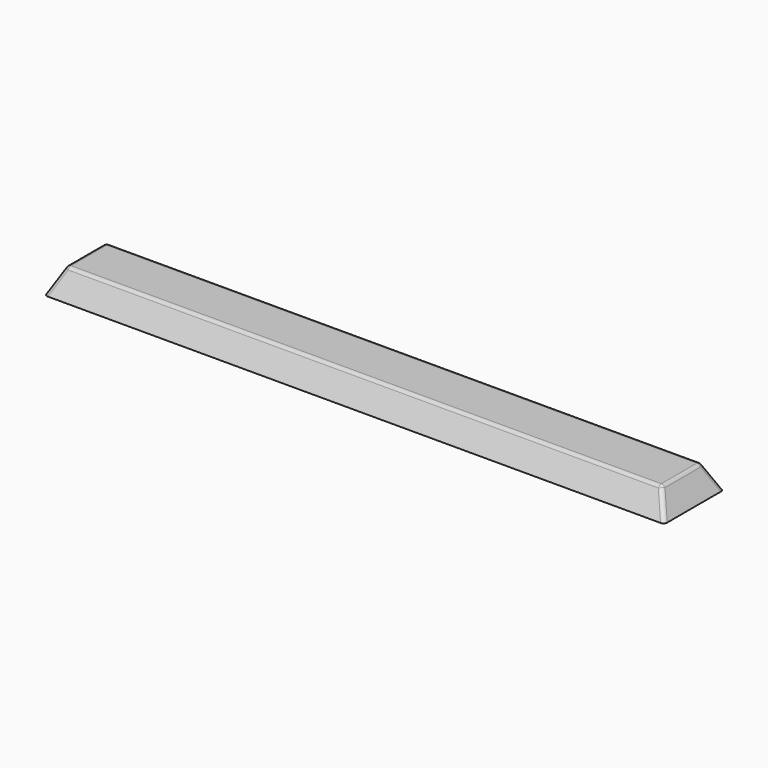
from build123d import *

# Parameters (mm, degrees)
F0_W        = 150
F0_H        = 18
F1_DEPTH    = 6
F2_T1_DEPTH = 49.0779464854
F2_T3_DEPTH = 181.0779464854
F3_R        = 1
F4_T        = -1.5
F5_R        = 2.8
F6_DEPTH    = 2.5
F7_W        = 1.5
F7_H        = 1.2
F7_W_2      = 1.2
F7_H_2      = 1.5
F8_DEPTH    = 2.5
F9_R        = 2.8
F10_DEPTH   = 2.5


# Not quite as in the source:
# - a fillet or chamfer that OpenCascade refuses, or shapes differently, is made with other operations: its cross-section is extruded or revolved along the edge and cut away or added


with BuildPart() as f1:
    # F0 (on Top) → F1 (new body)
    with BuildSketch(Plane.XY):
        Rectangle(F0_W, F0_H)
    extrude(amount=F1_DEPTH)

    # F2: chamfer of 3 x 6 on 4 edges, made by hand

    # F2_s2 → F2_t1 (cut)
    with BuildSketch(Plane.XZ.offset(-24.5389732427)):
        Polygon((75, 0), (72, 6), (75, 6), align=None)
        Polygon((-75, 0), (-72, 6), (-75, 6), align=None)
    extrude(amount=F2_T1_DEPTH, mode=Mode.SUBTRACT)

    # F2_s4 → F2_t3 (cut)
    with BuildSketch(Plane.YZ.offset(-90.5389732427)):
        Polygon((9, 0), (6, 6), (9, 6), align=None)
        Polygon((-9, 0), (-6, 6), (-9, 6), align=None)
    extrude(amount=F2_T3_DEPTH, mode=Mode.SUBTRACT)

    # F3
    f3_edges = [f1.edges().sort_by_distance(p)[0] for p in [
        (-73.5, 7.5, 3),
        (-73.5, -7.5, 3),
        (-72, 0, 6),
        (0, 6, 6),
        (72, 0, 6),
        (0, -6, 6),
        (73.5, 7.5, 3),
        (73.5, -7.5, 3),
    ]]
    fillet(f3_edges, radius=F3_R)

    # F4
    f4_openings = [f1.faces().sort_by_distance(p)[0] for p in [
        (0, 0, 0),
    ]]
    offset(amount=F4_T, openings=f4_openings)

    # F5 (on face) → F6 (join)
    with BuildSketch(Plane(origin=(0, 0, 4.5), x_dir=(1, 0, 0), z_dir=(0, 0, -1))):
        Circle(F5_R)
    extrude(amount=F6_DEPTH)

    # F7 (on face) → F8 (cut)
    with BuildSketch(Plane(origin=(0, 0, 2), x_dir=(1, 0, 0), z_dir=(0, 0, -1))):
        with Locations((-1.35, 0)):
            Rectangle(F7_W, F7_H)
        Rectangle(F7_W_2, F7_H)
        with Locations((0, -1.35)):
            Rectangle(F7_W_2, F7_H_2)
        with Locations((1.35, 0)):
            Rectangle(F7_W, F7_H)
        with Locations((0, 1.35)):
            Rectangle(F7_W_2, F7_H_2)
    extrude(amount=-F8_DEPTH, mode=Mode.SUBTRACT)

    # F9 (on face) → F10 (join)
    with BuildSketch(Plane(origin=(0, 0, 4.5), x_dir=(1, 0, 0), z_dir=(0, 0, -1))):
        with BuildLine():
            ThreePointArc((62.8, 0), (60, 2.8), (57.2, 0))
            ThreePointArc((57.2, 0), (60, -2.8), (62.8, 0))
        make_face()
        Polygon((57.9, -0.6), (57.9, 0), (57.9, 0.6), (59.4, 0.6), (59.4, 2.1), (60.6, 2.1), (60.6, 0.6), (62.1, 0.6), (62.1, -0.6), (60.6, -0.6), (60.6, -2.1), (59.4, -2.1), (59.4, -0.6), align=None, mode=Mode.SUBTRACT)
        with Locations((-60, 0)):
            Circle(F9_R)
        Polygon((-59.4, -0.6), (-59.4, -2.1), (-60.6, -2.1), (-60.6, -0.6), (-62.1, -0.6), (-62.1, 0.6), (-60.6, 0.6), (-60.6, 2.1), (-59.4, 2.1), (-59.4, 0.6), (-57.9, 0.6), (-57.9, -0.6), align=None, mode=Mode.SUBTRACT)
    extrude(amount=F10_DEPTH)


solid = f1.part
